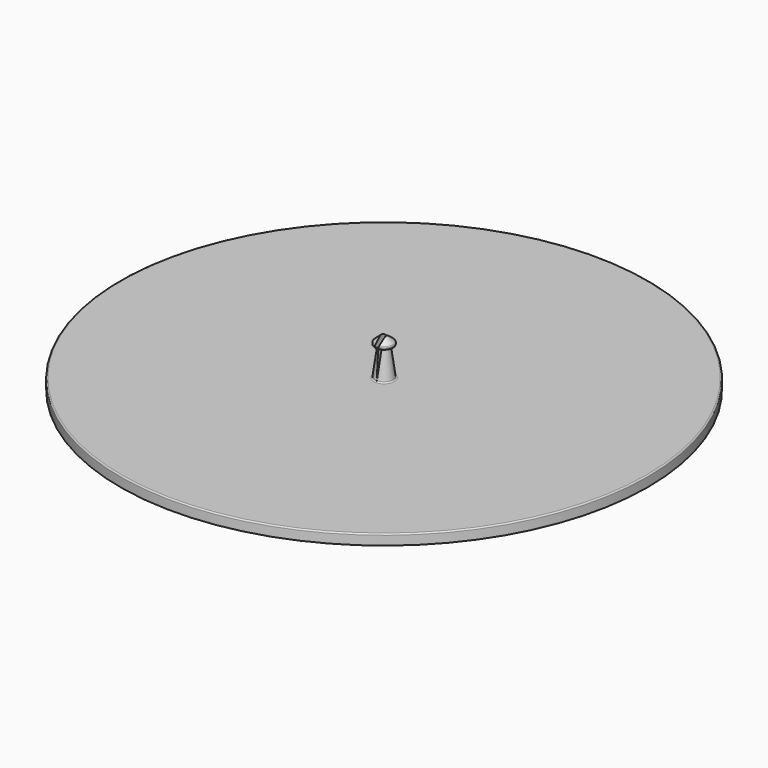
from build123d import *

# Parameters (mm, degrees)
F3_DEPTH      = 1000.001
F3_DEPTH_BACK = 1000.001
F4_T4_ANGLE   = 180
F4_T9_ANGLE   = 180
F4_T12_ANGLE  = 175.5397265939
F4_T14_ANGLE  = 175.5397265939
F4_T16_ANGLE  = 194.3823817652
F4_T18_ANGLE  = 194.3823817652


# Not quite as in the source:
# - a fillet or chamfer that OpenCascade refuses, or shapes differently, is made with other operations: its cross-section is extruded or revolved along the edge and cut away or added


with BuildPart() as f1:
    # F0 (on Front) → F1 (revolve)
    with BuildSketch(Plane.XZ):
        Polygon((0, 150), (0, 0), (35, 0), (20.1401172379, 107.9545454545), (35, 110), (35, 120), align=None)
        Polygon((35, 0), (0, 0), (0, -39.4391342998), (1000, -39.4391342998), (1000, 0), align=None)
    revolve(axis=Axis((0, 0, 75), (0, 0, -1)))

    # F2 (on Front) → F3 (cut, two sides)
    with BuildSketch(Plane.XZ) as f3_sk:
        Polygon((-9.2637268826, 157.2448909283), (0, 0), (9.2637268826, 157.2448909283), (0, 157.7906424325), align=None)
    extrude(amount=F3_DEPTH, mode=Mode.SUBTRACT)
    extrude(f3_sk.sketch, amount=-F3_DEPTH_BACK, mode=Mode.SUBTRACT)

    # F4: fillet of radius 5 on 7 edges, made by hand


with BuildPart() as f4_tool2:
    # F4_s3 → F4_t4 (revolve)
    with BuildSketch(Plane.YZ):
        with BuildLine():
            ThreePointArc((39.3588989435, 0), (36.0732552402, 1.2311081928), (34.4056046895, 4.3181818182))
            Line((34.4056046895, 4.3181818182), (35, 0))
            Line((35, 0), (39.3588989435, 0))
        make_face()
    revolve(axis=Axis((0, 0, 0), (0, 0, -1)), revolution_arc=F4_T4_ANGLE)

    split(bisect_by=Plane(origin=(0, 0, 0), x_dir=(0, 1, 0), z_dir=(0.9982691489, 0, -0.0588107677)), keep=Keep.TOP)


with BuildPart() as f1_1:
    add(f1.part)

    # F4_t1: union F4_tool2
    add(f4_tool2.part)


with BuildPart() as f4_tool7:
    # F4_s8 → F4_t9 (revolve)
    with BuildSketch(Plane.YZ):
        with BuildLine():
            ThreePointArc((-39.3588989435, 0), (-36.0732552402, 1.2311081928), (-34.4056046895, 4.3181818182))
            Line((-34.4056046895, 4.3181818182), (-35, 0))
            Line((-35, 0), (-39.3588989435, 0))
        make_face()
    revolve(axis=Axis((0, 0, 0), (0, 0, -1)), revolution_arc=F4_T9_ANGLE)

    split(bisect_by=Plane(origin=(0, 0, 0), x_dir=(0, 1, 0), z_dir=(-0.9982691489, 0, -0.0588107677)), keep=Keep.TOP)


with BuildPart() as f1_2:
    add(f1_1.part)

    # F4_t6: union F4_tool7
    add(f4_tool7.part)

    # F4_s11 → F4_t12 (revolve, cut)
    with BuildSketch(Plane(origin=(0, 0, 0), x_dir=(0, 0, 1), z_dir=(-0.9992425868, 0.0389134008, 0))):
        with BuildLine():
            ThreePointArc((121.4966083995, 33.2539568673), (119.7896094353, 34.5425644925), (117.7003253876, 35))
            Line((117.7003253876, 35), (120, 35))
            Line((120, 35), (121.4966083995, 33.2539568673))
        make_face()
    revolve(axis=Axis((0, 0, 120), (0, 0, -1)), revolution_arc=F4_T12_ANGLE, mode=Mode.SUBTRACT)

    # F4_s13 → F4_t14 (revolve, cut)
    with BuildSketch(Plane(origin=(0, 0, 0), x_dir=(0, 0, 1), z_dir=(0.9992425868, -0.0389134008, 0))):
        with BuildLine():
            ThreePointArc((117.7003253876, 35), (119.7896094353, 34.5425644925), (121.4966083995, 33.2539568673))
            Line((121.4966083995, 33.2539568673), (120, 35))
            Line((120, 35), (117.7003253876, 35))
        make_face()
    revolve(axis=Axis((0, 0, 120), (0, 0, -1)), revolution_arc=F4_T14_ANGLE, mode=Mode.SUBTRACT)

    # F4_s15 → F4_t16 (revolve, cut)
    with BuildSketch(Plane(origin=(0, 0, 0), x_dir=(0, 0, 1), z_dir=(0.9921339593, 0.1251806963, 0))):
        with BuildLine():
            ThreePointArc((109.4056046895, 30.6818181818), (111.0732552402, 33.7688918072), (114.3588989435, 35))
            Line((114.3588989435, 35), (110, 35))
            Line((110, 35), (109.4056046895, 30.6818181818))
        make_face()
    revolve(axis=Axis((0, 0, 110), (0, 0, -1)), revolution_arc=F4_T16_ANGLE, mode=Mode.SUBTRACT)

    # F4_s17 → F4_t18 (revolve, cut)
    with BuildSketch(Plane(origin=(0, 0, 0), x_dir=(0, 0, 1), z_dir=(-0.9921339593, -0.1251806963, 0))):
        with BuildLine():
            ThreePointArc((114.3588989435, 35), (111.0732552402, 33.7688918072), (109.4056046895, 30.6818181818))
            Line((109.4056046895, 30.6818181818), (110, 35))
            Line((110, 35), (114.3588989435, 35))
        make_face()
    revolve(axis=Axis((0, 0, 110), (0, 0, -1)), revolution_arc=F4_T18_ANGLE, mode=Mode.SUBTRACT)

    # F4_s19 → F4_t20 (revolve, cut)
    with BuildSketch(Plane.XZ):
        with BuildLine():
            ThreePointArc((1000, -5), (998.5355339059, -1.4644660941), (995, 0))
            Line((995, 0), (1000, 0))
            Line((1000, 0), (1000, -5))
        make_face()
    revolve(axis=Axis((0, 0, 0), (0, 0, -1)), mode=Mode.SUBTRACT)


solid = f1_2.part
